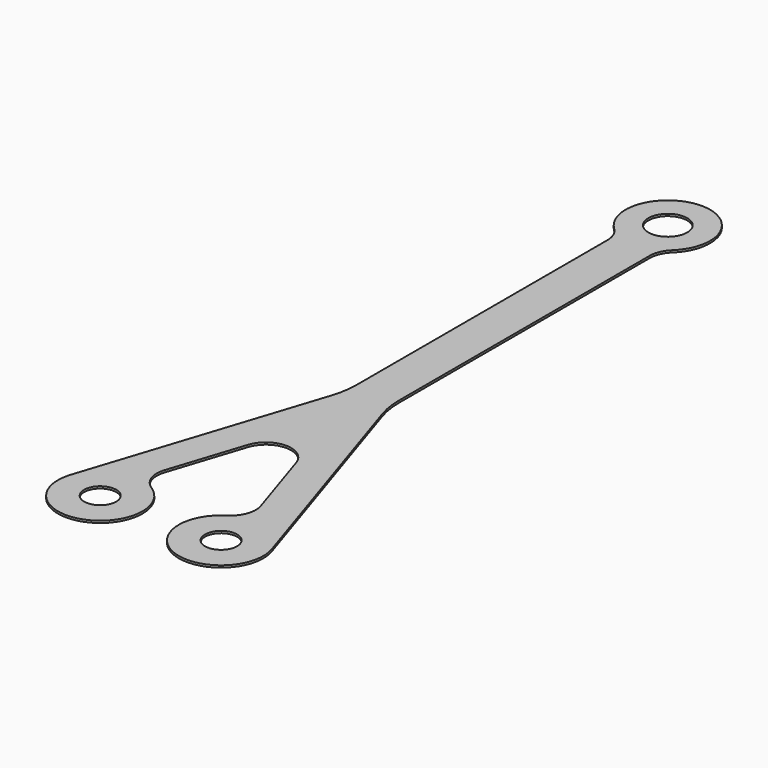
from build123d import *

# Parameters (mm, degrees)
F0_R     = 3.8
F0_R_2   = 4.6
F1_DEPTH = 0.5


# Not quite as in the source:
# - a feature names something its author has since deleted; it is built from what else it names


with BuildPart() as f1:
    # F0 (on Top) → F1 (new body)
    with BuildSketch(Plane.XY):
        with BuildLine():
            ThreePointArc((24.3621806055, 39.2965673213), (24.8508286843, 41.6682755665), (26.2371806055, 43.6536735858))
            ThreePointArc((26.2371806055, 43.6536735858), (19.3621806055, 60.91551736), (12.4871806055, 43.6536735858))
            ThreePointArc((12.4871806055, 43.6536735858), (13.8735325268, 41.6682755665), (14.3621806055, 39.2965673213))
            Line((14.3621806055, 39.2965673213), (14.3621806055, -34.8549244096))
            ThreePointArc((14.3621806055, -34.8549244096), (14.1166056215, -37.9794551404), (13.3859113767, -41.0272552129))
            Line((13.3859113767, -41.0272552129), (-4.4496847801, -95.9983172384))
            ThreePointArc((-4.4496847801, -95.9983172384), (8.4471568034, -108.4941551178), (10.428313753, -90.646199933))
            ThreePointArc((10.428313753, -90.646199933), (8.0021901548, -87.6142160275), (7.9408744101, -83.7315310678))
            Line((7.9408744101, -83.7315310678), (13.6550613742, -66.1198446814))
            ThreePointArc((13.6550613742, -66.1198446814), (19.3621806055, -61.9715439224), (25.0692998369, -66.1198446814))
            Line((25.0692998369, -66.1198446814), (30.783486801, -83.7315310678))
            ThreePointArc((30.783486801, -83.7315310678), (30.7221710563, -87.6142160275), (28.2960474581, -90.646199933))
            ThreePointArc((28.2960474581, -90.646199933), (30.2772044076, -108.4941551178), (43.1740459911, -95.9983172384))
            Line((43.1740459911, -95.9983172384), (25.3384498343, -41.0272552129))
            ThreePointArc((25.3384498343, -41.0272552129), (24.6077555896, -37.9794551404), (24.3621806055, -34.8549244096))
            Line((24.3621806055, -34.8549244096), (24.3621806055, 39.2965673213))
        make_face()
        with Locations((5.0621806055, -99.08448264)):
            Circle(F0_R, mode=Mode.SUBTRACT)
        with Locations((33.6621806055, -99.08448264)):
            Circle(F0_R, mode=Mode.SUBTRACT)
        with Locations((19.3621806055, 50.91551736)):
            Circle(F0_R_2, mode=Mode.SUBTRACT)
    extrude(amount=F1_DEPTH)


solid = f1.part
